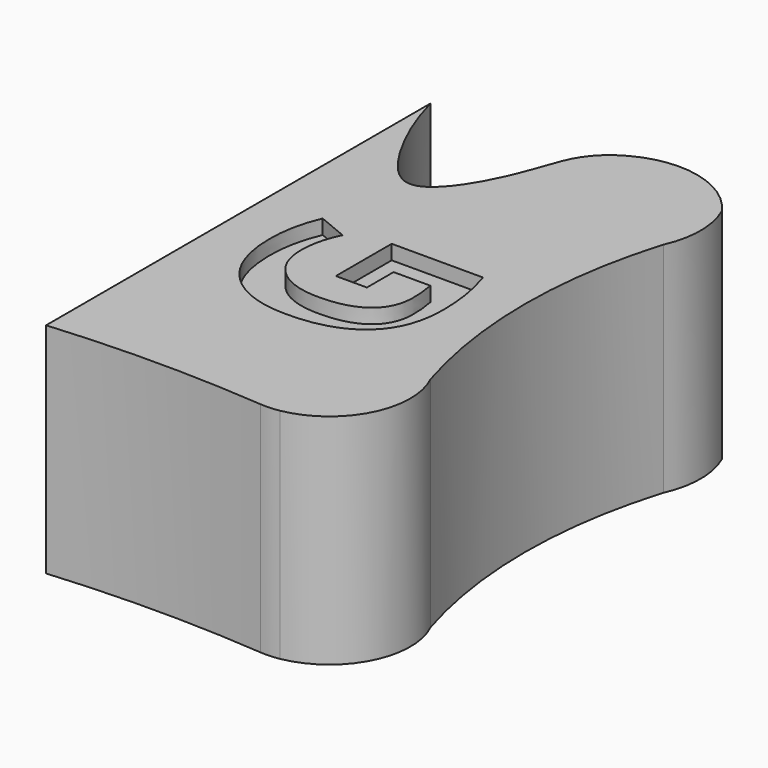
from build123d import *

# Parameters (mm, degrees)
F1_DEPTH     = 15
F2_TEXT_SIZE = 16.9274851223
F3_DEPTH     = 1
F6_ANGLE     = 270


# Not quite as in the source:
# - Text() gives the source's letters only with a copy of the font that has no kerning and outlines rounded to 1/6400 em; it was checked with that copy


with BuildPart() as f1:
    # F0 (on Top) → F1 (new body)
    with BuildSketch(Plane.XY):
        with BuildLine():
            add(Edge.make_bspline(
                [(-17.9661038518, 39.6488005223), (-17.5230307533, 37.9774820129), (-16.3472382307, 34.8607305267), (-12.9887485596, 30.1403988906), (-9.7132989598, 34.5500630667), (-8.8024825482, 37.4049689405), (-8.3030454209, 38.7657460461)],
                knots=[0, 0, 0, 0, 0.2648862461, 0.5, 0.7351137539, 0.9528188534, 0.9528188534, 0.9528188534, 0.9528188534], degree=3))
            Line((-17.9661038518, 39.6488005223), (-17.9661038518, 6.6488005223))
            ThreePointArc((-17.9661038518, 6.6488005223), (-10.6187071089, 6.9646587491), (-3.2702722389, 6.6739522346))
            ThreePointArc((-3.2702722389, 6.6739522346), (-2.6249586559, 6.6634932467), (-1.9836738105, 6.7362445898))
            ThreePointArc((-1.9836738105, 6.7362445898), (1.9936847169, 9.6929868794), (2.0338961482, 14.6488005223))
            ThreePointArc((2.0338961482, 14.6488005223), (0.5338961482, 24.6488005223), (2.0338961482, 34.6488005223))
            ThreePointArc((2.0338961482, 34.6488005223), (2.5716718659, 37.1488005223), (2.0338961482, 39.6488005223))
            ThreePointArc((2.0338961482, 39.6488005223), (-1.9339926598, 42.1609630146), (-6.5120941894, 41.1140206259))
            ThreePointArc((-6.5120941894, 41.1140206259), (-7.5849028886, 40.0751294043), (-8.3030454209, 38.7657460461))
        make_face()
    extrude(amount=F1_DEPTH)


with BuildPart() as f3:
    # F2 (on face) → F3 (new body)
    with BuildSketch(Plane.XY.offset(15)):
        with Locations((-14.7161038518, 14.6187304061)):
            Text('G', F2_TEXT_SIZE, font='Open Sans', font_style=FontStyle.BOLD, text_align=(TextAlign.LEFT, TextAlign.BOTTOM))
    extrude(amount=-F3_DEPTH)


with BuildPart() as f3_1:
    # F6: moved
    add(f3.part.rotate(Axis((-8.7161038518, 20.7126250501, 8.5332853347), (0, 0, -1)), F6_ANGLE))


with BuildPart() as f1_1:
    add(f1.part)

    # F7: cut F3
    add(f3_1.part, mode=Mode.SUBTRACT)


solid = f1_1.part
